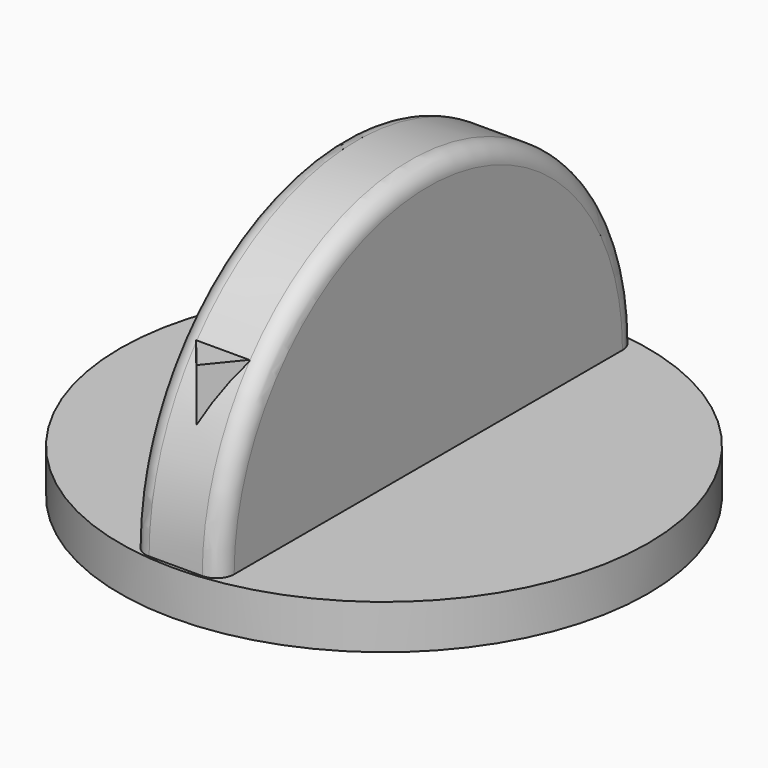
from build123d import *

# Parameters (mm, degrees)
F0_R          = 29.8
F1_DEPTH      = 5
F3_DEPTH      = 5
F3_DEPTH_BACK = 5
F5_DEPTH      = 20
F6_DEPTH      = 23.78
F7_T2_ANGLE   = 180
F7_T4_ANGLE   = 180


# Not quite as in the source:
# - a fillet or chamfer that OpenCascade refuses, or shapes differently, is made with other operations: its cross-section is extruded or revolved along the edge and cut away or added


with BuildPart() as f1:
    # F0 (on Top) → F1 (new body)
    with BuildSketch(Plane.XY):
        Circle(F0_R)
        Polygon((0, -26.4465436339), (-3, -22.7629262954), (0, -22.7629262954), (3, -22.7629262954), align=None, mode=Mode.SUBTRACT)
    extrude(amount=F1_DEPTH)

    # F2 (on Right) → F3 (join, two sides)
    with BuildSketch(Plane.YZ) as f3_sk:
        with BuildLine():
            Line((-29.4, 5), (29.4, 5))
            ThreePointArc((29.4, 5), (0, 34.4), (-29.4, 5))
        make_face()
    extrude(amount=-F3_DEPTH)
    extrude(f3_sk.sketch, amount=F3_DEPTH_BACK)

    # F4 (on Top) → F5 (cut)
    with BuildSketch(Plane.XY):
        with BuildLine():
            ThreePointArc((-3.0525563058, 1.38), (-0.7058457252, -3.2747949267), (3.35, 0))
            ThreePointArc((3.35, 0), (3.2747949267, 0.7058457252), (3.0525563058, 1.38))
            Line((3.0525563058, 1.38), (-3.0525563058, 1.38))
        make_face()
    extrude(amount=F5_DEPTH, mode=Mode.SUBTRACT)

    # F0 (on Top) → F6 (join)
    with BuildSketch(Plane.XY):
        Polygon((0, -22.7629262954), (-3, -22.7629262954), (0, -26.4465436339), (3, -22.7629262954), align=None)
    extrude(amount=F6_DEPTH)

    # F7: fillet of radius 2 on 2 edges, made by hand

    # F7_s1 → F7_t2 (revolve, cut)
    with BuildSketch(Plane.XY.offset(5)):
        with BuildLine():
            ThreePointArc((-3, 29.4), (-4.4142135624, 28.8142135624), (-5, 27.4))
            Line((-5, 27.4), (-5, 29.4))
            Line((-5, 29.4), (-3, 29.4))
        make_face()
    revolve(axis=Axis((-5, 0, 5), (1, 0, 0)), revolution_arc=F7_T2_ANGLE, mode=Mode.SUBTRACT)

    # F7_s3 → F7_t4 (revolve, cut)
    with BuildSketch(Plane.XY.offset(5)):
        with BuildLine():
            ThreePointArc((5, 27.4), (4.4142135624, 28.8142135624), (3, 29.4))
            Line((3, 29.4), (5, 29.4))
            Line((5, 29.4), (5, 27.4))
        make_face()
    revolve(axis=Axis((5, 0, 5), (1, 0, 0)), revolution_arc=F7_T4_ANGLE, mode=Mode.SUBTRACT)


solid = f1.part
